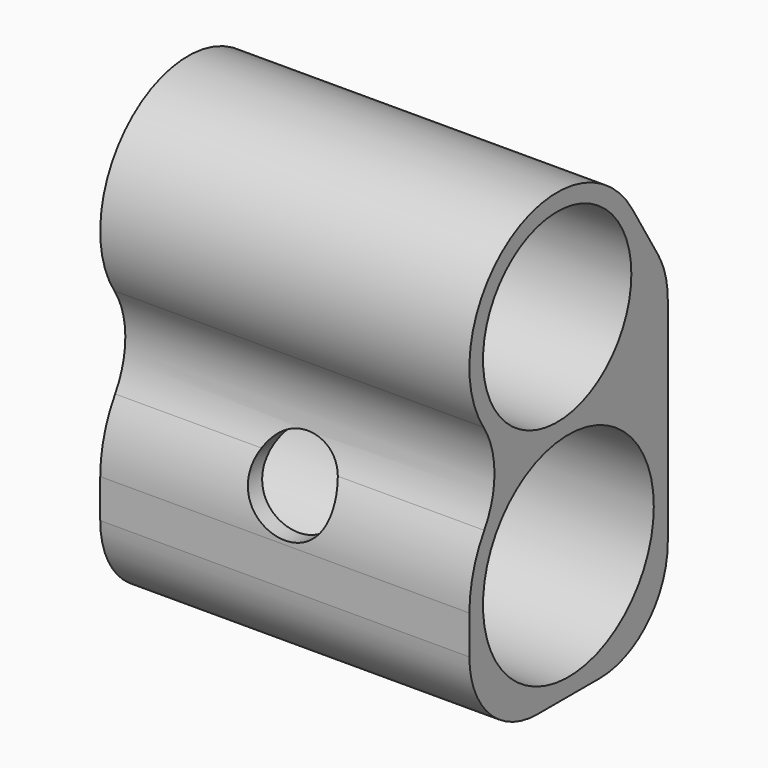
from build123d import *

# Parameters (mm, degrees)
F0_W          = 43.4
F0_H          = 38
F0_R          = 3
F1_DEPTH      = 2
F2_R          = 12.55
F2_R_2        = 10.9
F3_DEPTH      = 21.7
F3_DEPTH_BACK = 21.7
F4_R          = 5
F5_DEPTH      = 27.151
F8_R          = 10


# Not quite as in the source:
# - a feature names something its author has since deleted; it is built from what else it names


with BuildPart() as f1:
    # F0 (on Front) → F1 (new body)
    with BuildSketch(Plane.XZ):
        with Locations((0, -1)):
            Rectangle(F0_W, F0_H)
        Circle(F0_R, mode=Mode.SUBTRACT)
    extrude(amount=F1_DEPTH)

    # F2 (on Right) → F3 (join, two sides)
    with BuildSketch(Plane.YZ) as f3_sk:
        with BuildLine():
            ThreePointArc((-27.0737723252, 12.9281979258), (-25.4648034923, 7.5886797024), (-26.9655996144, 2.217753659))
            ThreePointArc((-26.9655996144, 2.217753659), (-28.5932479144, -1.4635839649), (-29.15, -5.45))
            Line((-29.15, -5.45), (-29.15, -20))
            Line((-29.15, -20), (-2, -20))
            Line((-2, -20), (-2, 18))
            Line((-2, 18), (0, 18))
            Line((0, 18), (-5.2100705327, 26.6195334989))
            ThreePointArc((-5.2100705327, 26.6195334989), (-23.0965208991, 30.8796696778), (-27.0737723252, 12.9281979258))
        make_face()
        with Locations((-14.6, -5.45)):
            Circle(F2_R, mode=Mode.SUBTRACT)
        with Locations((-16.25, 19.9464564457)):
            Circle(F2_R_2, mode=Mode.SUBTRACT)
    extrude(amount=-F3_DEPTH)
    extrude(f3_sk.sketch, amount=F3_DEPTH_BACK)

    # F4 (on face) → F5 (cut, through all)
    with BuildSketch(Plane(origin=(0, -2, 0), x_dir=(-1, 0, 0), z_dir=(0, 1, 0))):
        Circle(F4_R)
    extrude(amount=-F5_DEPTH, mode=Mode.SUBTRACT)

    # F6 (on Top) → F7 (revolve, cut)
    with BuildSketch(Plane.XY):
        Polygon((0, -2), (0, 0), (-3, 0), (-3, -0.3), (-5, -2), align=None)
    revolve(axis=Axis((0, -1, 0), (0, -1, 0)), mode=Mode.SUBTRACT)

    # F8
    f8_edges = [f1.edges().sort_by_distance(p)[0] for p in [
        (0, 0, -20),
        (0, 0, 18),
        (0, -29.15, -20),
    ]]
    fillet(f8_edges, radius=F8_R)


solid = f1.part
